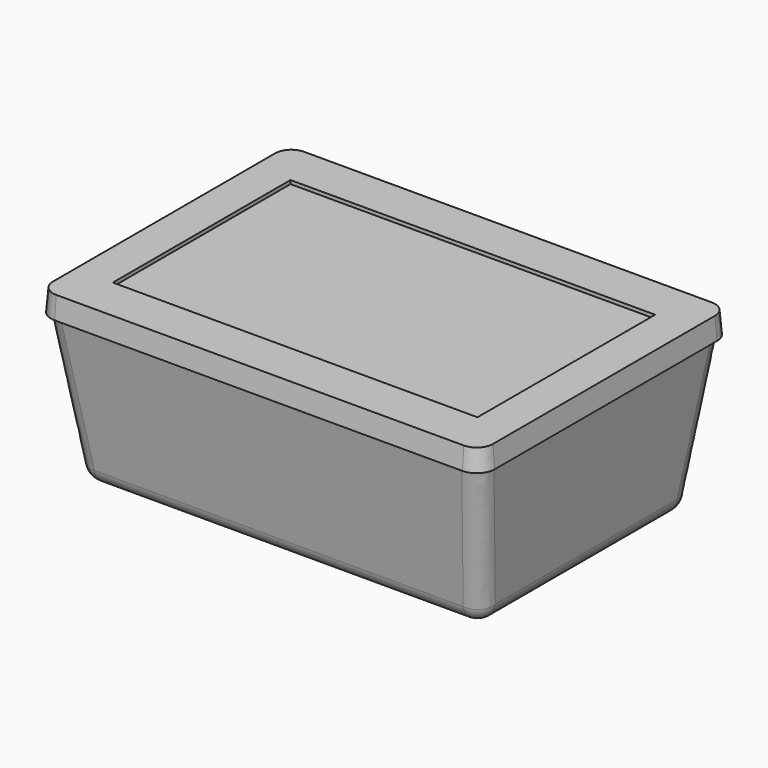
from build123d import *

# Parameters (mm, degrees)
F0_W      = 111.22
F0_H      = 71.63
F2_W      = 121.14
F2_H      = 85.07
F4_R      = 5
F5_W      = 123.14
F5_H      = 87.07
F6_DEPTH  = 6
F7_W      = 101.22
F7_H      = 61.63
F8_DEPTH  = 1
F9_R      = 5
F10_SIZE2 = 5.99999
F10_SIZE  = 0.524922


# Not quite as in the source:
# - a fillet or chamfer is up to 0.001 mm smaller than in the source, because OpenCascade refuses the exact size


with BuildPart() as f3:
    # F0 (on Top) → F3 section 0
    with BuildSketch(Plane.XY):
        Rectangle(F0_W, F0_H)
    # F2 (on offset) → F3 section 1
    with BuildSketch(Plane.XY.offset(42)):
        Rectangle(F2_W, F2_H)
    loft()

    # F4
    f4_edges = [f3.edges().sort_by_distance(p)[0] for p in [
        (-55.61, 0, 0),
        (-58.09, 39.175, 21),
        (0, 35.815, 0),
        (55.61, 0, 0),
        (58.09, 39.175, 21),
        (-58.09, -39.175, 21),
        (0, -35.815, 0),
        (58.09, -39.175, 21),
    ]]
    fillet(f4_edges, radius=F4_R)

    # F5 (on face) → F6 (join)
    with BuildSketch(Plane.XY.offset(42)):
        Rectangle(F5_W, F5_H)
        with BuildLine():
            Line((60.57, 37.5652286365), (60.57, -37.5652286365))
            add(Edge.make_bspline(
                [(60.57, -37.5652286365), (60.57, -37.8677629795), (60.5484249291, -38.1785474247), (60.5029654317, -38.4950915318), (60.4316524162, -38.8141360023), (60.3333363666, -39.1316751054), (60.0821499269, -39.7565973164), (59.9290553292, -40.0639382754), (59.7486936762, -40.3612591505), (59.5421641644, -40.6440796366), (59.3119172372, -40.9083408285), (58.8238966802, -41.3807158702), (58.5682195509, -41.5910650721), (58.2970619174, -41.7793580892), (58.013945443, -41.9437291503), (57.7226574277, -42.0834034649), (57.1273207787, -42.3149957608), (56.8231561933, -42.4063160322), (56.5180078096, -42.4725842951), (56.2153860403, -42.5148862736), (55.9181609136, -42.535), (55.628544141, -42.535)],
                knots=[0, 0, 0, 0, 0, 0, 0, 0.2552622354, 0.2552622354, 0.2552622354, 0.2552622354, 0.2552622354, 0.5115672797, 0.5115672797, 0.5115672797, 0.5115672797, 0.5115672797, 0.7543107062, 0.7543107062, 0.7543107062, 0.7543107062, 0.7543107062, 1, 1, 1, 1, 1, 1, 1], degree=6))
            Line((55.628544141, -42.535), (-55.628544141, -42.535))
            add(Edge.make_bspline(
                [(-60.57, -37.5652286365), (-60.57, -37.8677629794), (-60.5484249292, -38.1785474246), (-60.5029654317, -38.4950915316), (-60.4316524163, -38.814136002), (-60.3333363667, -39.1316751051), (-60.0821499271, -39.756597316), (-59.9290553294, -40.0639382751), (-59.7486936764, -40.3612591501), (-59.5421641646, -40.6440796363), (-59.3119172375, -40.9083408282), (-58.8238966804, -41.38071587), (-58.5682195512, -41.591065072), (-58.2970619176, -41.7793580891), (-58.0139454431, -41.9437291502), (-57.7226574278, -42.0834034648), (-57.1273207787, -42.3149957608), (-56.8231561933, -42.4063160322), (-56.5180078096, -42.4725842951), (-56.2153860403, -42.5148862736), (-55.9181609136, -42.535), (-55.628544141, -42.535)],
                knots=[0, 0, 0, 0, 0, 0, 0, 0.2552622353, 0.2552622353, 0.2552622353, 0.2552622353, 0.2552622353, 0.5115672797, 0.5115672797, 0.5115672797, 0.5115672797, 0.5115672797, 0.7543107062, 0.7543107062, 0.7543107062, 0.7543107062, 0.7543107062, 1, 1, 1, 1, 1, 1, 1], degree=6))
            Line((-60.57, -37.5652286365), (-60.57, 37.5652286365))
            add(Edge.make_bspline(
                [(-55.628544141, 42.535), (-55.9165579294, 42.535), (-56.2120960387, 42.5151083241), (-56.5129833201, 42.4732846379), (-56.8164007689, 42.4077788273), (-57.1189028719, 42.3175153178), (-57.7138767296, 42.0875473103), (-58.0063798227, 41.9479897602), (-58.2907253957, 41.7835490477), (-58.5630840084, 41.5949938834), (-58.8198912965, 41.3842007295), (-59.3081604347, 40.9123831651), (-59.5378156039, 40.6494264179), (-59.7439719788, 40.3680131083), (-59.924197311, 40.0721470067), (-60.0773872558, 39.7662523131), (-60.3304237584, 39.1410513034), (-60.4299622755, 38.821673494), (-60.5021575431, 38.500700594), (-60.5481693204, 38.1822186305), (-60.57, 37.8695496868), (-60.57, 37.5652286365)],
                knots=[0, 0, 0, 0, 0, 0, 0, 0.2443294294, 0.2443294294, 0.2443294294, 0.2443294294, 0.2443294294, 0.4879249993, 0.4879249993, 0.4879249993, 0.4879249993, 0.4879249993, 0.7432302237, 0.7432302237, 0.7432302237, 0.7432302237, 0.7432302237, 1, 1, 1, 1, 1, 1, 1], degree=6))
            Line((-55.628544141, 42.535), (55.628544141, 42.535))
            add(Edge.make_bspline(
                [(60.57, 37.5652286365), (60.57, 37.8677629794), (60.5484249292, 38.1785474246), (60.5029654317, 38.4950915316), (60.4316524163, 38.814136002), (60.3333363667, 39.1316751051), (60.0821499271, 39.756597316), (59.9290553294, 40.0639382751), (59.7486936764, 40.3612591501), (59.5421641646, 40.6440796363), (59.3119172375, 40.9083408282), (58.8238966804, 41.38071587), (58.5682195512, 41.591065072), (58.2970619176, 41.7793580891), (58.0139454431, 41.9437291502), (57.7226574278, 42.0834034648), (57.1273207787, 42.3149957608), (56.8231561933, 42.4063160322), (56.5180078096, 42.4725842951), (56.2153860403, 42.5148862736), (55.9181609136, 42.535), (55.628544141, 42.535)],
                knots=[0, 0, 0, 0, 0, 0, 0, 0.2552622353, 0.2552622353, 0.2552622353, 0.2552622353, 0.2552622353, 0.5115672797, 0.5115672797, 0.5115672797, 0.5115672797, 0.5115672797, 0.7543107062, 0.7543107062, 0.7543107062, 0.7543107062, 0.7543107062, 1, 1, 1, 1, 1, 1, 1], degree=6))
        make_face(mode=Mode.SUBTRACT)
        with BuildLine():
            add(Edge.make_bspline(
                [(60.57, -37.5652286365), (60.57, -37.8677629795), (60.5484249291, -38.1785474247), (60.5029654317, -38.4950915318), (60.4316524162, -38.8141360023), (60.3333363666, -39.1316751054), (60.0821499269, -39.7565973164), (59.9290553292, -40.0639382754), (59.7486936762, -40.3612591505), (59.5421641644, -40.6440796366), (59.3119172372, -40.9083408285), (58.8238966802, -41.3807158702), (58.5682195509, -41.5910650721), (58.2970619174, -41.7793580892), (58.013945443, -41.9437291503), (57.7226574277, -42.0834034649), (57.1273207787, -42.3149957608), (56.8231561933, -42.4063160322), (56.5180078096, -42.4725842951), (56.2153860403, -42.5148862736), (55.9181609136, -42.535), (55.628544141, -42.535)],
                knots=[0, 0, 0, 0, 0, 0, 0, 0.2552622354, 0.2552622354, 0.2552622354, 0.2552622354, 0.2552622354, 0.5115672797, 0.5115672797, 0.5115672797, 0.5115672797, 0.5115672797, 0.7543107062, 0.7543107062, 0.7543107062, 0.7543107062, 0.7543107062, 1, 1, 1, 1, 1, 1, 1], degree=6))
            Line((60.57, -37.5652286365), (60.57, 37.5652286365))
            add(Edge.make_bspline(
                [(60.57, 37.5652286365), (60.57, 37.8677629794), (60.5484249292, 38.1785474246), (60.5029654317, 38.4950915316), (60.4316524163, 38.814136002), (60.3333363667, 39.1316751051), (60.0821499271, 39.756597316), (59.9290553294, 40.0639382751), (59.7486936764, 40.3612591501), (59.5421641646, 40.6440796363), (59.3119172375, 40.9083408282), (58.8238966804, 41.38071587), (58.5682195512, 41.591065072), (58.2970619176, 41.7793580891), (58.0139454431, 41.9437291502), (57.7226574278, 42.0834034648), (57.1273207787, 42.3149957608), (56.8231561933, 42.4063160322), (56.5180078096, 42.4725842951), (56.2153860403, 42.5148862736), (55.9181609136, 42.535), (55.628544141, 42.535)],
                knots=[0, 0, 0, 0, 0, 0, 0, 0.2552622353, 0.2552622353, 0.2552622353, 0.2552622353, 0.2552622353, 0.5115672797, 0.5115672797, 0.5115672797, 0.5115672797, 0.5115672797, 0.7543107062, 0.7543107062, 0.7543107062, 0.7543107062, 0.7543107062, 1, 1, 1, 1, 1, 1, 1], degree=6))
            Line((55.628544141, 42.535), (-55.628544141, 42.535))
            add(Edge.make_bspline(
                [(-55.628544141, 42.535), (-55.9165579294, 42.535), (-56.2120960387, 42.5151083241), (-56.5129833201, 42.4732846379), (-56.8164007689, 42.4077788273), (-57.1189028719, 42.3175153178), (-57.7138767296, 42.0875473103), (-58.0063798227, 41.9479897602), (-58.2907253957, 41.7835490477), (-58.5630840084, 41.5949938834), (-58.8198912965, 41.3842007295), (-59.3081604347, 40.9123831651), (-59.5378156039, 40.6494264179), (-59.7439719788, 40.3680131083), (-59.924197311, 40.0721470067), (-60.0773872558, 39.7662523131), (-60.3304237584, 39.1410513034), (-60.4299622755, 38.821673494), (-60.5021575431, 38.500700594), (-60.5481693204, 38.1822186305), (-60.57, 37.8695496868), (-60.57, 37.5652286365)],
                knots=[0, 0, 0, 0, 0, 0, 0, 0.2443294294, 0.2443294294, 0.2443294294, 0.2443294294, 0.2443294294, 0.4879249993, 0.4879249993, 0.4879249993, 0.4879249993, 0.4879249993, 0.7432302237, 0.7432302237, 0.7432302237, 0.7432302237, 0.7432302237, 1, 1, 1, 1, 1, 1, 1], degree=6))
            Line((-60.57, 37.5652286365), (-60.57, -37.5652286365))
            add(Edge.make_bspline(
                [(-60.57, -37.5652286365), (-60.57, -37.8677629794), (-60.5484249292, -38.1785474246), (-60.5029654317, -38.4950915316), (-60.4316524163, -38.814136002), (-60.3333363667, -39.1316751051), (-60.0821499271, -39.756597316), (-59.9290553294, -40.0639382751), (-59.7486936764, -40.3612591501), (-59.5421641646, -40.6440796363), (-59.3119172375, -40.9083408282), (-58.8238966804, -41.38071587), (-58.5682195512, -41.591065072), (-58.2970619176, -41.7793580891), (-58.0139454431, -41.9437291502), (-57.7226574278, -42.0834034648), (-57.1273207787, -42.3149957608), (-56.8231561933, -42.4063160322), (-56.5180078096, -42.4725842951), (-56.2153860403, -42.5148862736), (-55.9181609136, -42.535), (-55.628544141, -42.535)],
                knots=[0, 0, 0, 0, 0, 0, 0, 0.2552622353, 0.2552622353, 0.2552622353, 0.2552622353, 0.2552622353, 0.5115672797, 0.5115672797, 0.5115672797, 0.5115672797, 0.5115672797, 0.7543107062, 0.7543107062, 0.7543107062, 0.7543107062, 0.7543107062, 1, 1, 1, 1, 1, 1, 1], degree=6))
            Line((-55.628544141, -42.535), (55.628544141, -42.535))
        make_face()
    extrude(amount=F6_DEPTH)

    # F7 (on face) → F8 (cut)
    with BuildSketch(Plane.XY.offset(48)):
        Rectangle(F7_W, F7_H)
    extrude(amount=-F8_DEPTH, mode=Mode.SUBTRACT)

    # F9
    f9_edges = [f3.edges().sort_by_distance(p)[0] for p in [
        (-61.57, 43.535, 45),
        (-61.57, -43.535, 45),
        (61.57, -43.535, 45),
        (61.57, 43.535, 45),
    ]]
    fillet(f9_edges, radius=F9_R)

    # F10 (size 0.5249319812 and 6 in the source; OpenCascade refuses exactly that, so slightly less here)
    f10_edges = [f3.edges().sort_by_distance(p)[0] for p in [
        (61.57, 0, 48),
        (60.105534, 42.070534, 48),
        (0, 43.535, 48),
        (-60.105534, 42.070534, 48),
        (-61.57, 0, 48),
        (-60.105534, -42.070534, 48),
        (0, -43.535, 48),
        (60.105534, -42.070534, 48),
    ]]
    f10_side = f3.faces().sort_by_distance((60.061867, 0, 48))[0]
    chamfer(f10_edges, length=F10_SIZE, length2=F10_SIZE2, reference=f10_side)


solid = f3.part
